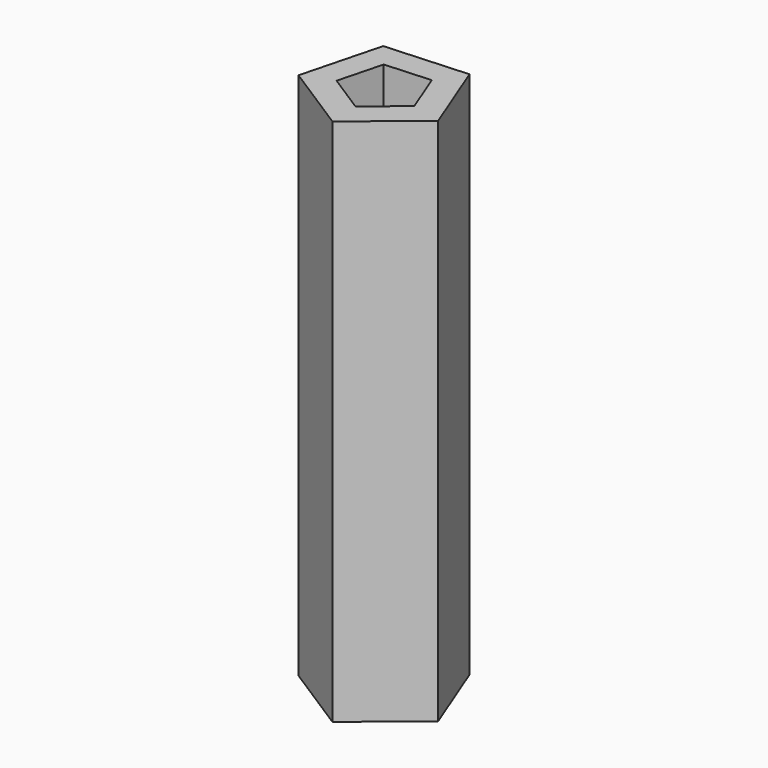
from build123d import *

# Parameters (mm, degrees)
F1_DEPTH = 177.8
F2_T     = -8.4666666667


# Not quite as in the source:
# - a length typed as a fraction of an inch, garbled in the dataset ("3 / 203.2 mm" for 3/8 in), is restored


with BuildPart() as f1:
    # F0 (on Top) → F1 (new body)
    with BuildSketch(Plane.XY):
        Polygon((-35.4204343678, -8.8066042373), (-13.96876778, 8.8066042373), (-24.0909949393, 34.6511322751), (-51.7985419534, 33.0107205511), (-58.8005205937, 6.1523623123), align=None)
    extrude(amount=F1_DEPTH)

    # F2
    f2_openings = [f1.faces().sort_by_distance(p)[0] for p in [
        (-36.815852, 14.762843, 177.8),
    ]]
    offset(amount=F2_T, openings=f2_openings)


solid = f1.part
